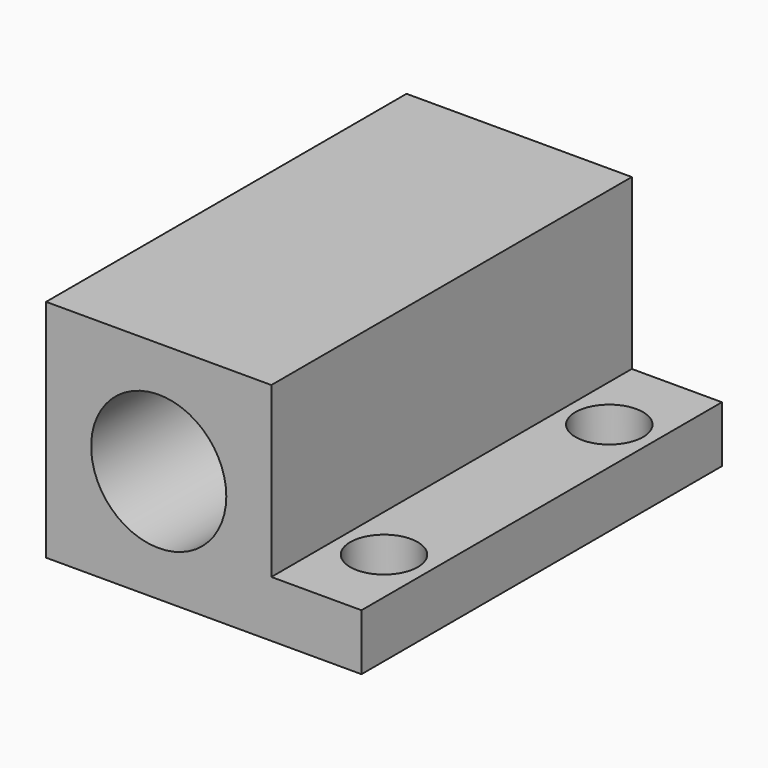
from build123d import *
from build123d import SkipClean  # not in build123d's __all__

# Parameters (mm, degrees)
F0_W     = 28
F0_H     = 40
F1_DEPTH = 5
F2_W     = 20
F2_H     = 40
F3_DEPTH = 15
F6_D     = 6
F4_R     = 6
F7_DEPTH = 25
F8_R     = 6
F9_DEPTH = 16


with BuildPart() as f1:
    # F0 (on Top) → F1 (new body)
    with BuildSketch(Plane.XY):
        with Locations((14, 20)):
            Rectangle(F0_W, F0_H)
    extrude(amount=F1_DEPTH)

    # F2 (on face) → F3 (join)
    with BuildSketch(Plane.XY.offset(5)):
        with Locations((10, 20)):
            Rectangle(F2_W, F2_H)
    extrude(amount=F3_DEPTH)

    # F6 (through all)
    with Locations(Plane.XY.offset(5)):
        with Locations((24, 32.5), (24, 7.5)):
            Hole(F6_D / 2)

    # F4 (on face) → F7 (cut)
    with BuildSketch(Plane.XZ):
        with Locations((10, 10)):
            Circle(F4_R)
    extrude(amount=-F7_DEPTH, mode=Mode.SUBTRACT)

    # F8 (on face) → F9 (cut)
    with BuildSketch(Plane(origin=(0, 0, 0), x_dir=(1, 0, 0), z_dir=(0, 0, -1))):
        with Locations((10, -25)):
            Circle(F8_R)
    with SkipClean():  # cleaning this boolean's faces spoils the solid; the shape is the same uncleaned
        extrude(amount=-F9_DEPTH, mode=Mode.SUBTRACT)


solid = f1.part
